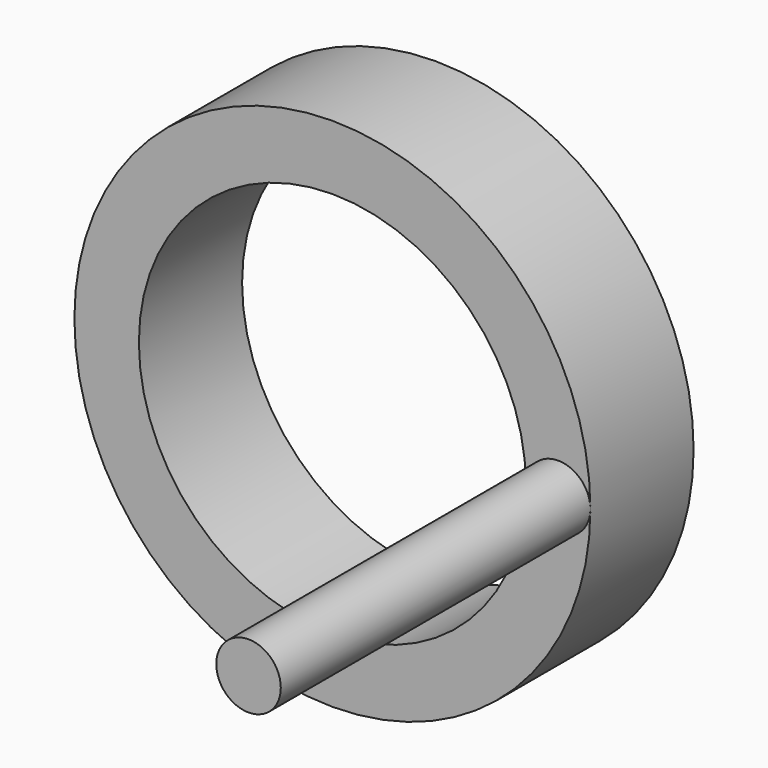
from build123d import *

# Parameters (mm, degrees)
F0_R     = 25.4
F0_R_2   = 19.05
F1_DEPTH = 6.35
F3_DEPTH = 38.1


with BuildPart() as f1:
    # F0 (on Front) → F1 (new body, symmetric)
    with BuildSketch(Plane.XZ):
        with Locations((-25.4, 25.4)):
            Circle(F0_R)
        with Locations((-25.4, 25.4)):
            Circle(F0_R_2, mode=Mode.SUBTRACT)
    extrude(amount=F1_DEPTH, both=True)

    # F2 (on face) → F3 (join)
    with BuildSketch(Plane.XZ.offset(6.35)):
        with BuildLine():
            ThreePointArc((-6.35, 25.4), (-3.175, 22.225), (0, 25.4))
            ThreePointArc((0, 25.4), (-3.175, 28.575), (-6.35, 25.4))
        make_face()
    extrude(amount=F3_DEPTH)


solid = f1.part
